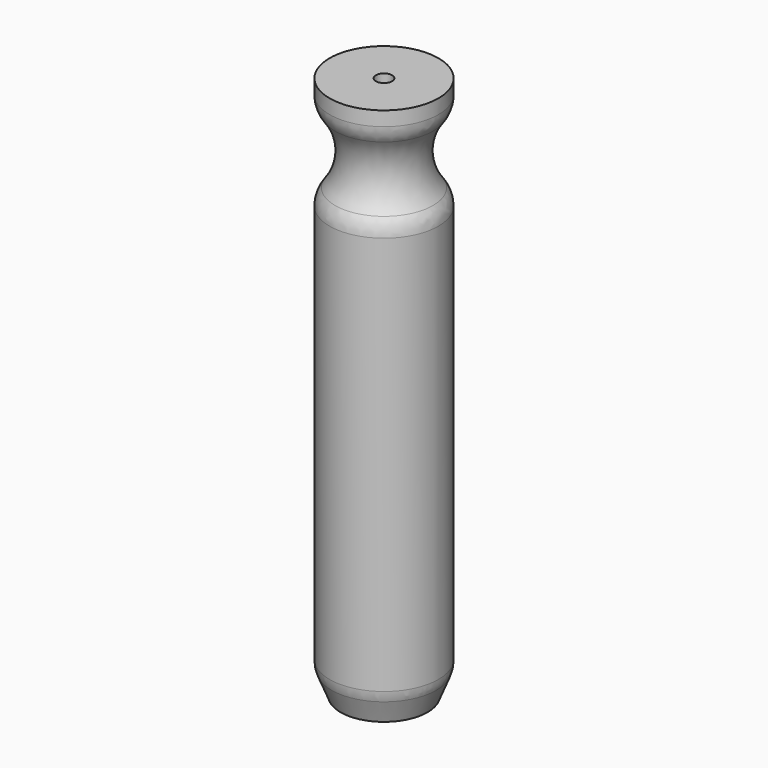
from build123d import *

# Parameters (mm, degrees)
F2_R     = 10
F3_DEPTH = 100
F4_SIZE2 = 2
F4_SIZE  = 5
F5_R     = 1.5
F6_DEPTH = 50
F9_R     = 5
F10_R    = 5


# Not quite as in the source:
# - two fillets or chamfers of one size are made in one step


with BuildPart() as f3:
    # F2 (on Top) → F3 (new body)
    with BuildSketch(Plane.XY):
        Circle(F2_R)
    extrude(amount=F3_DEPTH)

    # F4
    f4_edges = [f3.edges().sort_by_distance(p)[0] for p in [
        (-10, 0, 0),
    ]]
    f4_side = f3.faces().sort_by_distance((-10, 0, 50))[0]
    chamfer(f4_edges, length=F4_SIZE, length2=F4_SIZE2, reference=f4_side)

    # F5 (on face) → F6 (cut)
    with BuildSketch(Plane.XY.offset(100)):
        Circle(F5_R)
    extrude(amount=-F6_DEPTH, mode=Mode.SUBTRACT)

    # F7 (on Front) → F8 (revolve, cut)
    with BuildSketch(Plane.XZ):
        with BuildLine():
            Line((13.1810711939, 79.0897459622), (13.1810711939, 97.5897459622))
            ThreePointArc((13.1810711939, 97.5897459622), (6.9807422323, 88.3397459622), (13.1810711939, 79.0897459622))
        make_face()
    revolve(axis=Axis((0, 0, 50), (0, 0, -1)), mode=Mode.SUBTRACT)

    # F9
    f9_edges = [f3.edges().sort_by_distance(p)[0] for p in [
        (-10, 0, 81.179492),
    ]]
    fillet(f9_edges, radius=F9_R)

    # F10
    f10_edges = [f3.edges().sort_by_distance(p)[0] for p in [
        (-10, 0, 5),
        (-10, 0, 95.5),
    ]]
    fillet(f10_edges, radius=F10_R)


solid = f3.part
